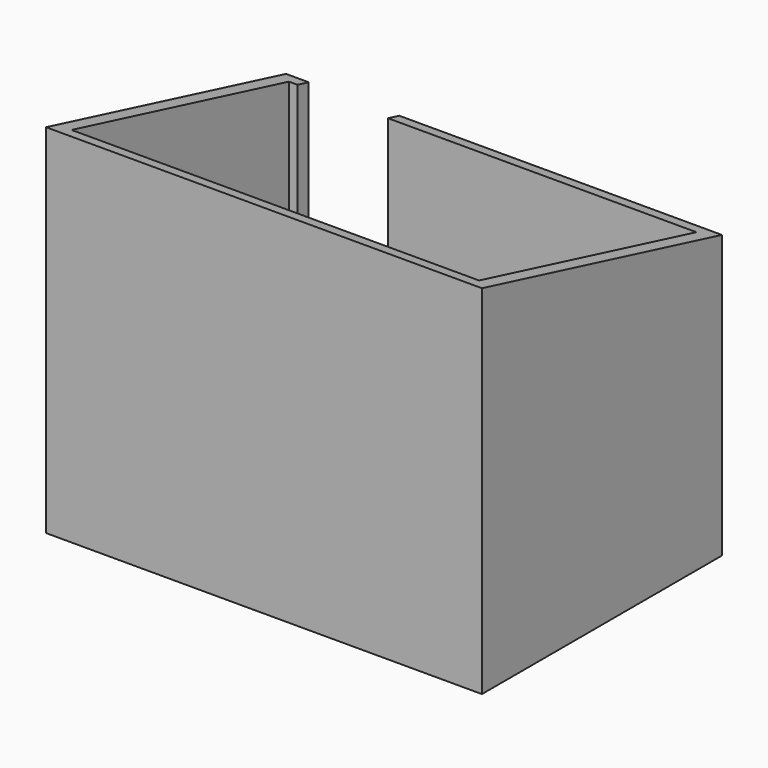
from build123d import *

# Parameters (mm, degrees)
F3_REACH = 7828.3953141922
F4_W     = 3911.6
F4_H     = 2692.4
F5_DEPTH = 127


with BuildPart() as f3:
    f3_end = Plane(origin=(0, 717.1764705882, 2868.7058823529), x_dir=(0, 0.9701425001, -0.242535625), z_dir=(0, 0.242535625, 0.9701425001))
    # F0 (on Top) → F3 (new body, up to a plane its end follows)
    with BuildSketch(Plane.XY):
        Polygon((3657.6, 0), (0, 0), (0, 2438.4), (76.2, 2438.4), (76.2, 2565.4), (-127, 2565.4), (-127, -127), (3784.6, -127), (3784.6, 2565.4), (889, 2565.4), (889, 2438.4), (3657.6, 2438.4), align=None)
    f3_long = extrude(amount=F3_REACH, mode=Mode.PRIVATE)
    add(split(f3_long, bisect_by=f3_end, keep=Keep.BOTTOM, mode=Mode.PRIVATE))

    # F4 (on face) → F5 (join)
    with BuildSketch(Plane(origin=(0, 0, 0), x_dir=(1, 0, 0), z_dir=(0, 0, -1))):
        with Locations((1828.8, -1219.2)):
            Rectangle(F4_W, F4_H)
    extrude(amount=F5_DEPTH)


solid = f3.part
